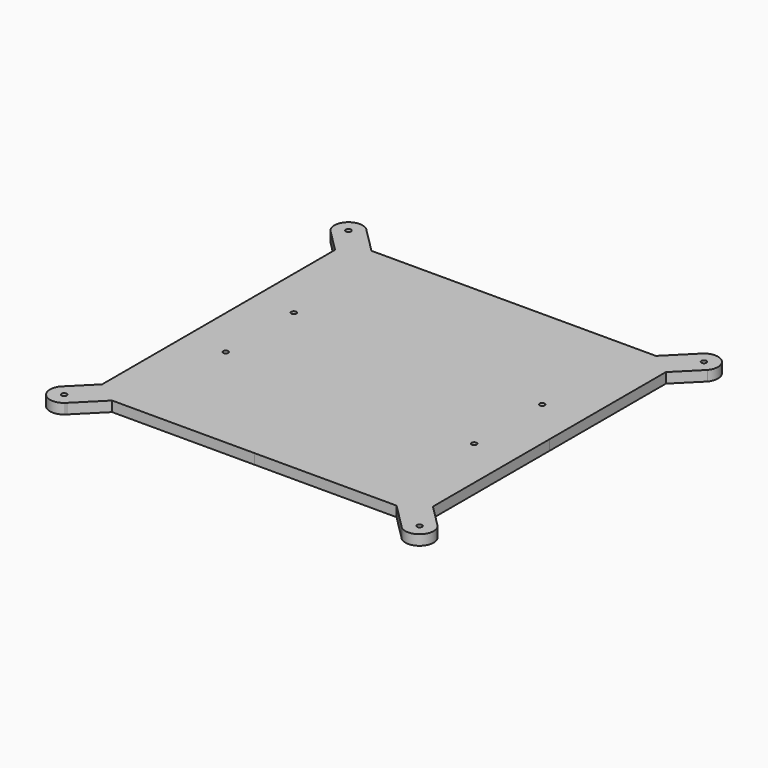
from build123d import *

# Parameters (mm, degrees)
F0_R     = 1.5098129389
F0_R_2   = 1.5
F1_DEPTH = 6


# Not quite as in the source:
# - ends of sketch curves that miss each other by under 0.0002 mm in the source are joined


with BuildPart() as f1:
    # F0 (on Top) → F1 (new body)
    with BuildSketch(Plane.XY):
        with BuildLine():
            Line((4.5e-05, 95.32702), (-83.6431340024, 95.32702))
            Line((-83.6431340024, 95.32702), (-98.2850169252, 109.9708148351))
            Line((-98.2850169252, 109.9708148351), (-99.0283260424, 110.7142210123))
            ThreePointArc((-99.0283260424, 110.7142210123), (-110.2653878227, 110.4426468905), (-110.8769341282, 99.2189522637))
            Line((-110.8769341282, 99.2189522637), (-97.25943, 85.599669985))
            Line((-97.25943, 85.599669985), (-97.25943, -2.5e-06))
            Line((-97.25943, -2.5e-06), (-97.2594255995, -85.5996749849))
            Line((-97.2594255995, -85.5996749849), (-110.8769290275, -99.2189579637))
            ThreePointArc((-110.8769290275, -99.2189579637), (-110.2653821451, -110.4426525591), (-99.0283203508, -110.7142261032))
            Line((-99.0283203508, -110.7142261032), (-98.2850112718, -109.9708198877))
            Line((-98.2850112718, -109.9708198877), (-83.6431291018, -95.3270243))
            Line((-83.6431291018, -95.3270243), (4.99006e-05, -95.32702))
            Line((4.99006e-05, -95.32702), (83.6432191018, -95.3270243))
            Line((83.6432191018, -95.3270243), (98.2851012718, -109.9708198877))
            Line((98.2851012718, -109.9708198877), (99.0284103508, -110.7142261032))
            ThreePointArc((99.0284103508, -110.7142261032), (110.2654721451, -110.4426525591), (110.8770190275, -99.2189579637))
            Line((110.8770190275, -99.2189579637), (97.2595155995, -85.5996749849))
            Line((97.2595155995, -85.5996749849), (97.25952, -2.5e-06))
            Line((97.25952, -2.5e-06), (97.25952, 85.599669985))
            Line((97.25952, 85.599669985), (110.8770241282, 99.2189522637))
            ThreePointArc((110.8770241282, 99.2189522637), (110.2654778227, 110.4426468905), (99.0284160424, 110.7142210123))
            Line((99.0284160424, 110.7142210123), (98.2851069252, 109.9708148351))
            Line((98.2851069252, 109.9708148351), (83.6432240024, 95.32702))
            Line((83.6432240024, 95.32702), (4.5e-05, 95.32702))
        make_face()
        with Locations((-104.4999496278, -104.5000026861)):
            Circle(F0_R, mode=Mode.SUBTRACT)
        with Locations((-73.0099637148, -25.0000018767)):
            Circle(F0_R_2, mode=Mode.SUBTRACT)
        with Locations((104.5000396278, -104.5000026861)):
            Circle(F0_R, mode=Mode.SUBTRACT)
        with Locations((73.0100537148, -25.0000018767)):
            Circle(F0_R_2, mode=Mode.SUBTRACT)
        with Locations((-73.009965, 24.9999981233)):
            Circle(F0_R_2, mode=Mode.SUBTRACT)
        with Locations((-104.499955, 104.4999973139)):
            Circle(F0_R, mode=Mode.SUBTRACT)
        with Locations((73.010055, 24.9999981233)):
            Circle(F0_R_2, mode=Mode.SUBTRACT)
        with Locations((104.500045, 104.4999973139)):
            Circle(F0_R, mode=Mode.SUBTRACT)
        with BuildLine():
            Line((-99.0283260424, 110.7142210123), (-98.2850169252, 109.9708148351))
            ThreePointArc((-98.2850169252, 109.9708148351), (-98.6448610267, 110.3543268389), (-99.0283260424, 110.7142210123))
        make_face()
        with BuildLine():
            ThreePointArc((99.0284160424, 110.7142210123), (98.6449510267, 110.3543268389), (98.2851069252, 109.9708148351))
            Line((98.2851069252, 109.9708148351), (99.0284160424, 110.7142210123))
        make_face()
        with BuildLine():
            Line((-98.2850112718, -109.9708198877), (-99.0283203508, -110.7142261032))
            ThreePointArc((-99.0283203508, -110.7142261032), (-98.6448553535, -110.35433191), (-98.2850112718, -109.9708198877))
        make_face()
        with BuildLine():
            ThreePointArc((98.2851012718, -109.9708198877), (98.6449453535, -110.35433191), (99.0284103508, -110.7142261032))
            Line((99.0284103508, -110.7142261032), (98.2851012718, -109.9708198877))
        make_face()
    extrude(amount=F1_DEPTH)


solid = f1.part
